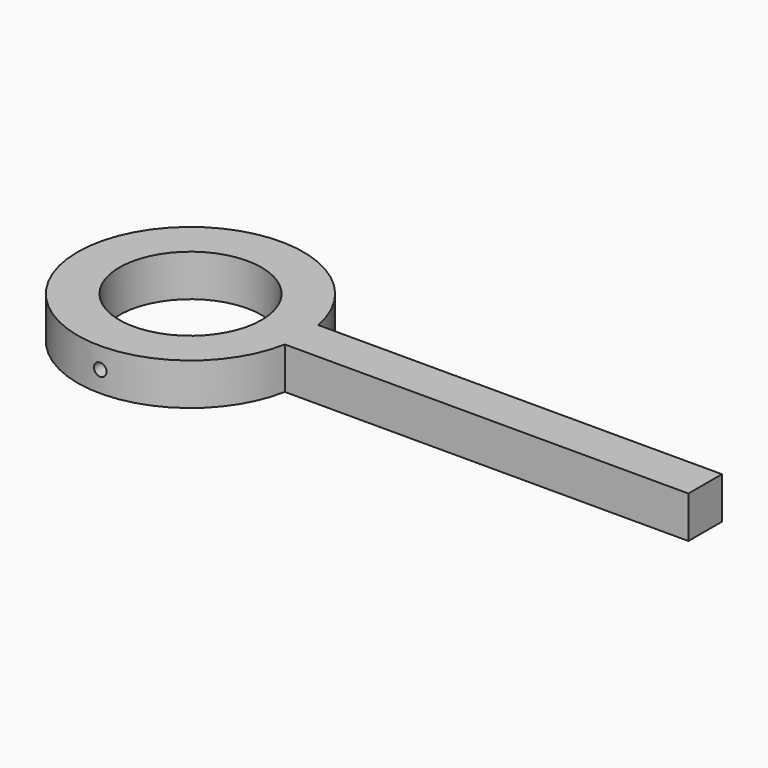
from build123d import *

# Parameters (mm, degrees)
F0_W     = 254
F0_H     = 254
F3_W     = 2540
F3_H     = 254
F4_DEPTH = 127
F6_DEPTH = 685.801


# Not quite as in the source:
# - a feature names something its author has since deleted; it is built from what else it names


with BuildPart() as f2:
    # F0 (on Front) → F2 (revolve)
    with BuildSketch(Plane.XZ):
        with Locations((558.8, 127)):
            Rectangle(F0_W, F0_H)
    revolve(axis=Axis((0, 0, 38.9041751623), (0, 0, 1)))

    # F3 (on Front) → F4 (join, symmetric)
    with BuildSketch(Plane.XZ):
        with Locations((1854.2, 127)):
            Rectangle(F3_W, F3_H)
    extrude(amount=F4_DEPTH, both=True)

    # F5 (on Front) → F6 (cut, through all)
    with BuildSketch(Plane.XZ):
        with BuildLine():
            ThreePointArc((0, 88.9), (26.9407683632, 100.0592316368), (38.1, 127))
            ThreePointArc((38.1, 127), (-26.9407683632, 153.9407683632), (0, 88.9))
        make_face()
    extrude(amount=F6_DEPTH, mode=Mode.SUBTRACT)


solid = f2.part
